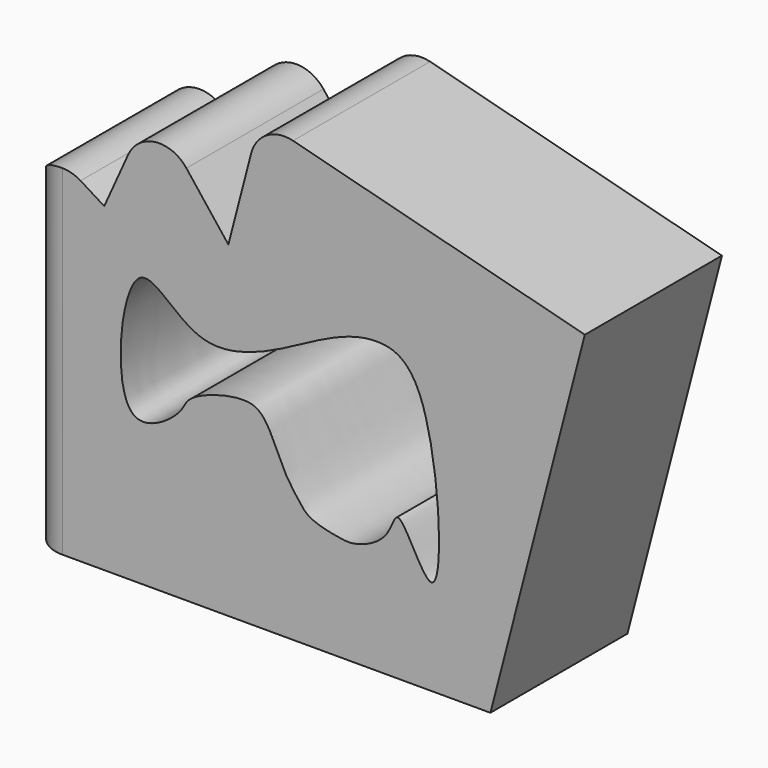
from build123d import *

# Parameters (mm, degrees)
F1_DEPTH = 25.4
F2_R     = 5.08
F4_DEPTH = 25.4


with BuildPart() as f1:
    # F0 (on Front) → F1 (new body)
    with BuildSketch(Plane.XZ):
        Polygon((-33.3446450531, 29.0814004838), (-44.6117855608, 36.0853001475), (-44.6117855608, -18.4232965112), (23.9046085626, -18.4232965112), (37.9123985767, 35.4762636125), (-10.2708584407, 47.9984612881), (-14.9353733665, 30.0502123182), (-26.3407472521, 44.6117855608), align=None)
    extrude(amount=F1_DEPTH)

    # F2
    f2_edges = [f1.edges().sort_by_distance(p)[0] for p in [
        (-26.340747, -12.7, 44.611786),
        (-10.270858, -12.7, 47.998461),
        (-44.611786, -12.7, 36.0853),
        (-44.611786, -25.4, 8.831002),
    ]]
    fillet(f2_edges, radius=F2_R)

    # F3 (on face) → F4 (cut)
    with BuildSketch(Plane.XZ.offset(25.4)):
        with BuildLine():
            add(Edge.make_bspline(
                [(13.4458132088, 19.6956638247), (11.74177874, 23.8300496783), (6.7957187469, 25.4028744107), (-1.9807003124, 22.3049317252), (-18.9071758323, 11.5463276334), (-30.0881670737, 29.3445522935), (-32.8799181246, -2.0787929379), (-21.6915838982, 5.5168211689), (-21.3106596952, 7.9917435161), (-17.1471336221, 9.9459320622), (-12.3205443457, 10.8171874288), (-9.7242920208, 9.7329395204), (-7.8552380833, 5.9205949814), (-6.5742563999, 2.8146495514), (-4.4723437738, -0.0344728039), (-2.9318667739, -1.9818520668), (1.5435597025, -2.9238525321), (4.0702578631, -3.154721813), (9.0494277088, -0.9396378917), (10.1039499737, 5.6404859645), (17.7927477883, -14.4493846447), (16.3712653316, 12.5978332976), (13.4458132088, 19.6956638247)],
                knots=[0, 0, 0, 0, 0.0564290034, 0.1166446169, 0.2000319696, 0.2636943375, 0.3474840522, 0.4002730146, 0.4325501392, 0.4729809081, 0.516868137, 0.5482718229, 0.587911654, 0.6251726423, 0.661589246, 0.6926096381, 0.7334052397, 0.7658304164, 0.8113742078, 0.846236586, 0.9031238213, 1, 1, 1, 1], degree=3))
        make_face()
    extrude(amount=-F4_DEPTH, mode=Mode.SUBTRACT)


solid = f1.part
